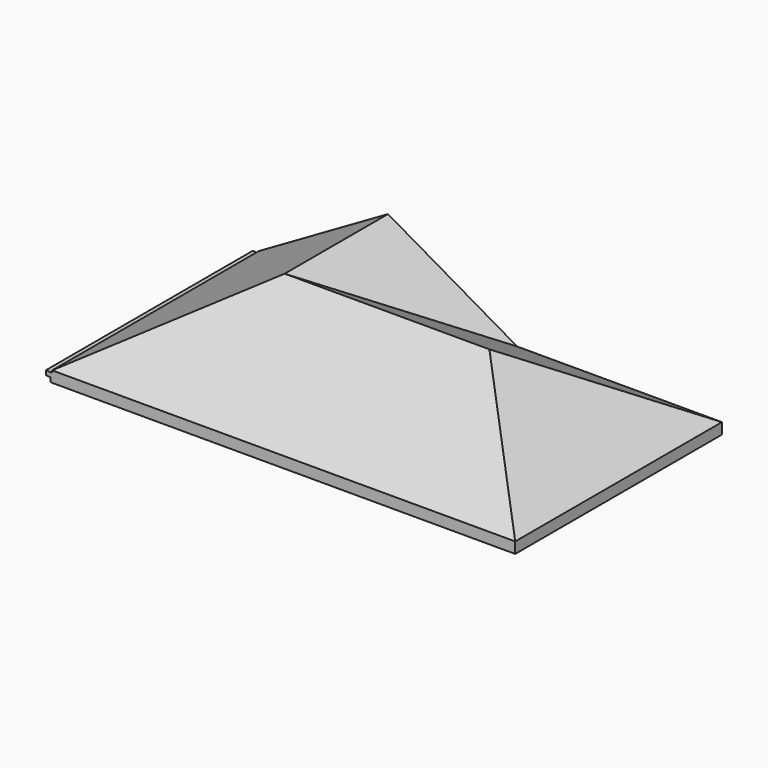
from build123d import *

# Parameters (mm, degrees)
F1_DEPTH = 10715
F3_DEPTH = 5978.001
F6_W     = 5978
F6_H     = 200
F7_DEPTH = 40
F9_DEPTH = 5978


with BuildPart() as f1:
    # F0 (on Right) → F1 (new body)
    with BuildSketch(Plane.YZ):
        Polygon((0, 255), (0, 0), (5978, 0), (5978, 255), (2989, 1980.6999546078), align=None)
    extrude(amount=F1_DEPTH)

    # F2 (on Front) → F3 (cut, through all)
    with BuildSketch(Plane.XZ):
        Polygon((0, 1980.6999546078), (0, 255), (2989, 1980.6999546078), align=None)
        Polygon((7726, 1980.6999546078), (10715, 255), (10715, 1980.6999546078), align=None)
    extrude(amount=-F3_DEPTH, mode=Mode.SUBTRACT)

    # F4 (on face) → F5 (join, up to the next surface of F1)
    with BuildSketch(Plane(origin=(0, 5978, 0), x_dir=(-1, 0, 0), z_dir=(0, 1, 0))):
        Polygon((-5978, 255), (0, 255), (-2989, 1980.6999546078), align=None)
    extrude(until=Until.NEXT, dir=(0, -1, 0))

    # F6 (on face) → F7 (join)
    with BuildSketch(Plane(origin=(0, 0, 0), x_dir=(0, -1, 0), z_dir=(-1, 0, 0))):
        with Locations((-2989, 105)):
            Rectangle(F6_W, F6_H)
    extrude(amount=F7_DEPTH)

    # F8 (on face) → F9 (join, through all)
    with BuildSketch(Plane(origin=(0, 5978, 0), x_dir=(-1, 0, 0), z_dir=(0, 1, 0))):
        Polygon((140, 215), (40, 205), (40, 105), (140, 105), align=None)
    extrude(amount=-F9_DEPTH)


solid = f1.part
